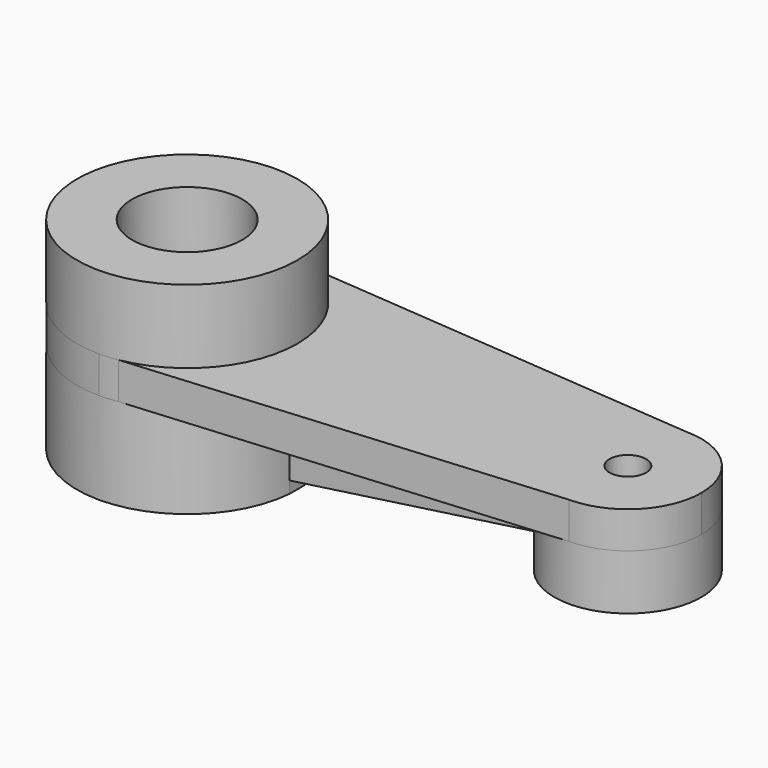
from build123d import *
from build123d import SkipClean  # not in build123d's __all__

# Parameters (mm, degrees)
F1_DEPTH  = 1.5875
F2_R      = 4.7625
F2_R_2    = 2.38125
F3_DEPTH  = 3.175
F4_R      = 4.7625
F4_R_2    = 2.38125
F5_DEPTH  = 3.96875
F6_R      = 3.175
F6_R_2    = 0.79375
F7_DEPTH  = 2.38125
F9_DEPTH  = 3.96875
F11_DEPTH = 25.4


with BuildPart() as f1:
    # F0 (on Top) → F1 (new body)
    with BuildSketch(Plane.XY):
        with BuildLine():
            Line((0.7882758621, 4.6968103448), (0, 4.7625))
            ThreePointArc((0, 4.7625), (-4.7625, 0), (0, -4.7625))
            Line((0, -4.7625), (0.7882758621, -4.6968103448))
            ThreePointArc((0.7882758621, -4.6968103448), (3.6356271841, -3.076299925), (4.7625, 0))
            ThreePointArc((4.7625, 0), (3.6356271841, 3.076299925), (0.7882758621, 4.6968103448))
        make_face()
        with BuildLine():
            ThreePointArc((2.38125, 0), (1.6837980227, -1.6837980227), (0, -2.38125))
            ThreePointArc((0, -2.38125), (-1.6837980227, 1.6837980227), (2.38125, 0))
        make_face(mode=Mode.SUBTRACT)
        with BuildLine():
            ThreePointArc((0.7882758621, 4.6968103448), (0.3955040978, 4.7460491736), (0, 4.7625))
            Line((0, 4.7625), (0.7882758621, 4.6968103448))
        make_face()
        with BuildLine():
            Line((0.7882758621, -4.6968103448), (0, -4.7625))
            ThreePointArc((0, -4.7625), (0.3955040978, -4.7460491736), (0.7882758621, -4.6968103448))
        make_face()
        with BuildLine():
            Line((19.05, 3.175), (0.7882758621, 4.6968103448))
            ThreePointArc((0.7882758621, 4.6968103448), (3.6356271841, 3.076299925), (4.7625, 0))
            ThreePointArc((4.7625, 0), (3.6356271841, -3.076299925), (0.7882758621, -4.6968103448))
            Line((0.7882758621, -4.6968103448), (19.05, -3.175))
            ThreePointArc((19.05, -3.175), (15.875, 0), (19.05, 3.175))
        make_face()
        with BuildLine():
            ThreePointArc((22.225, 0), (21.2950640303, 2.2450640303), (19.05, 3.175))
            ThreePointArc((19.05, 3.175), (15.875, 0), (19.05, -3.175))
            ThreePointArc((19.05, -3.175), (21.2950640303, -2.2450640303), (22.225, 0))
        make_face()
        with BuildLine():
            ThreePointArc((19.84375, 0), (19.6112660076, -0.5612660076), (19.05, -0.79375))
            ThreePointArc((19.05, -0.79375), (18.4887339924, 0.5612660076), (19.84375, 0))
        make_face(mode=Mode.SUBTRACT)
    extrude(amount=F1_DEPTH)

    # F2 (on face) → F3 (join)
    with BuildSketch(Plane.XY.offset(1.5875)):
        Circle(F2_R)
        Circle(F2_R_2, mode=Mode.SUBTRACT)
    with SkipClean():  # cleaning this boolean's faces spoils the solid; the shape is the same uncleaned
        extrude(amount=F3_DEPTH)

    # F4 (on face) → F5 (join)
    with BuildSketch(Plane(origin=(0, 0, 0), x_dir=(1, 0, 0), z_dir=(0, 0, -1))):
        Circle(F4_R)
        Circle(F4_R_2, mode=Mode.SUBTRACT)
    extrude(amount=F5_DEPTH)

    # F6 (on face) → F7 (join)
    with BuildSketch(Plane(origin=(0, 0, 0), x_dir=(1, 0, 0), z_dir=(0, 0, -1))):
        with Locations((19.05, 0)):
            Circle(F6_R)
        with Locations((19.05, 0)):
            Circle(F6_R_2, mode=Mode.SUBTRACT)
    extrude(amount=F7_DEPTH)

    # F8 (on face) → F9 (join, through all)
    with BuildSketch(Plane(origin=(0, 0, -3.96875), x_dir=(1, 0, 0), z_dir=(0, 0, -1))):
        with BuildLine():
            ThreePointArc((4.7459347324, 0.396875), (4.758356881, 0.1986102803), (4.7625, 0))
            ThreePointArc((4.7625, 0), (4.758356881, -0.1986102803), (4.7459347324, -0.396875))
            Line((4.7459347324, -0.396875), (15.8999023453, -0.396875))
            ThreePointArc((15.8999023453, -0.396875), (15.875, 0), (15.8999023453, 0.396875))
            Line((15.8999023453, 0.396875), (4.7459347324, 0.396875))
        make_face()
    extrude(amount=-F9_DEPTH)

    # F10 (on face) → F11 (cut)
    with BuildSketch(Plane(origin=(0, 0.396875, 0), x_dir=(-1, 0, 0), z_dir=(0, 1, 0))):
        Polygon((-4.7459347324, -3.96875), (-4.7459347324, -3.46075), (-15.8999023453, -1.87325), (-15.8999023453, -2.38125), (-15.8999023453, -3.96875), align=None)
    extrude(amount=-F11_DEPTH, mode=Mode.SUBTRACT)


solid = f1.part
